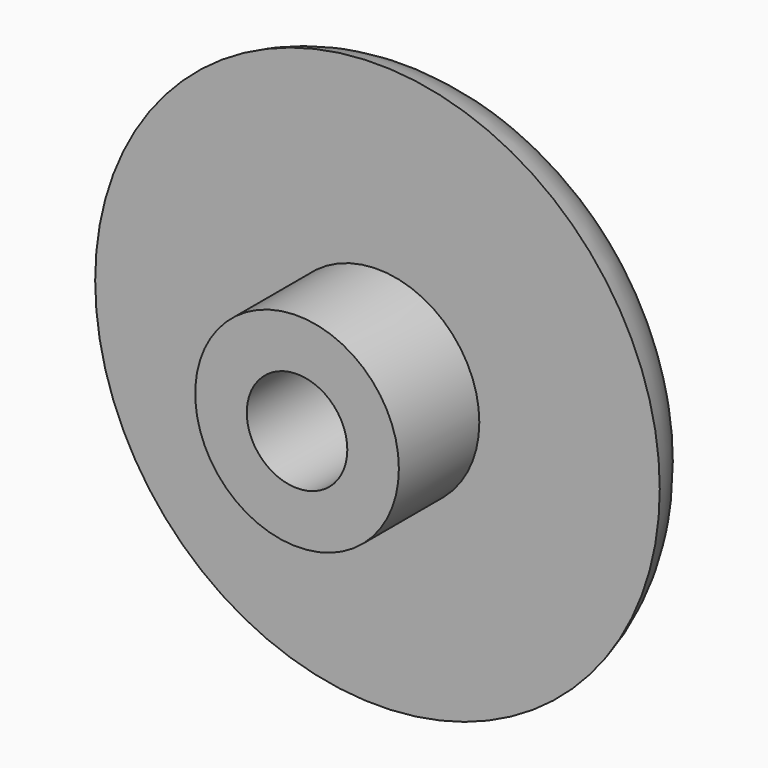
from build123d import *

# Parameters (mm, degrees)
F0_R     = 10.95
F1_DEPTH = 3
F2_R     = 3.95
F3_DEPTH = 6.9
F4_T     = -2


# Not quite as in the source:
# - a fillet or chamfer that OpenCascade refuses, or shapes differently, is made with other operations: its cross-section is extruded or revolved along the edge and cut away or added


with BuildPart() as f1:
    # F0 (on Front) → F1 (new body)
    with BuildSketch(Plane.XZ):
        Circle(F0_R)
    extrude(amount=F1_DEPTH)

    # F2 (on Front) → F3 (join)
    with BuildSketch(Plane.XZ):
        Circle(F2_R)
    extrude(amount=F3_DEPTH)

    # F4
    f4_openings = [f1.faces().sort_by_distance(p)[0] for p in [
        (0, -6.9, 0),
    ]]
    offset(amount=F4_T, openings=f4_openings, kind=Kind.INTERSECTION)

    # F5: fillet of radius 3.81 on 1 edges, made by hand

    # F5_s1 → F5_t2 (revolve, cut)
    with BuildSketch(Plane.XY):
        with BuildLine():
            ThreePointArc((10.95, -3), (9.6177045238, -0.843335206), (7.2270979062, 0))
            Line((7.2270979062, 0), (10.95, 0))
            Line((10.95, 0), (10.95, -3))
        make_face()
    revolve(axis=Axis((0, 0, 0), (0, -1, 0)), mode=Mode.SUBTRACT)


solid = f1.part
